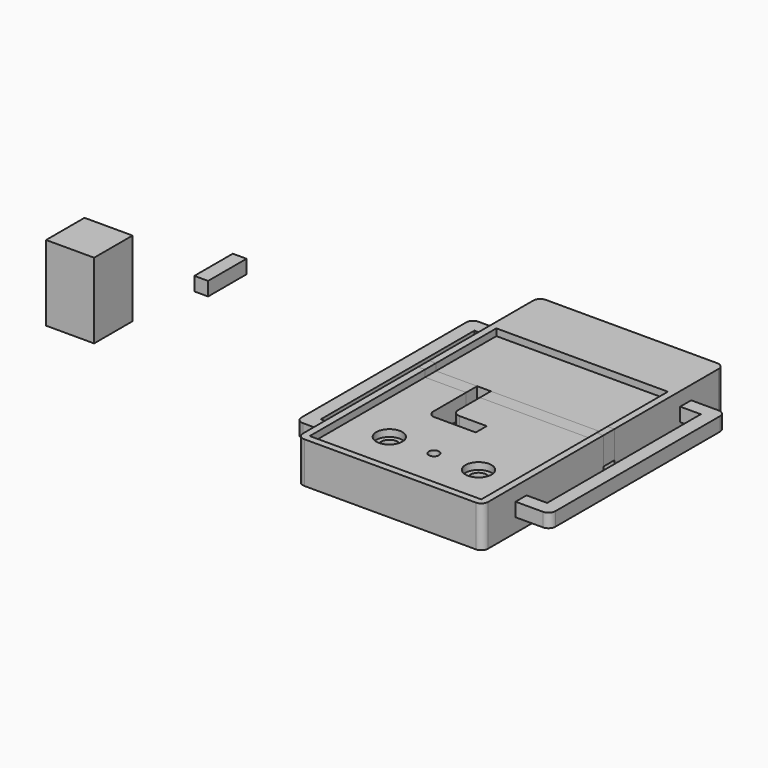
from build123d import *

# Parameters (mm, degrees)
F1_DEPTH  = 6
F0_R      = 1.9
F0_R_2    = 0.75
F2_DEPTH  = 5
F3_START  = 2
F3_DEPTH  = 2
F4_START  = 2
F0_W      = 1
F0_H      = 2
F4_DEPTH  = 4
F5_START  = 2.5
F0_W_2    = 6
F5_DEPTH  = 2.5
F0_W_3    = 17
F6_DEPTH  = 2
F0_R_3    = 1.2
F7_DEPTH  = 4
F8_W      = 2
F8_H      = 7
F9_DEPTH  = 2
F8_W_2    = 7
F10_DEPTH = 9


with BuildPart() as f1:
    # F0 (on Top) → F1 (new body)
    with BuildSketch(Plane.XY):
        with BuildLine():
            Line((12.5, 0), (0, 0))
            Line((0, 0), (-12.5, 0))
            Line((-12.5, 0), (-12.5, 21))
            Line((-12.5, 21), (-13.5, 21))
            Line((-13.5, 21), (-13.5, 7))
            Line((-13.5, 7), (-13.5, 5))
            Line((-13.5, 5), (-13.5, 0))
            ThreePointArc((-13.5, 0), (-13.2071067812, -0.7071067812), (-12.5, -1))
            Line((-12.5, -1), (0, -1))
            Line((0, -1), (12.5, -1))
            ThreePointArc((12.5, -1), (13.2071067812, -0.7071067812), (13.5, 0))
            Line((13.5, 0), (13.5, 5))
            Line((13.5, 5), (13.5, 7))
            Line((13.5, 7), (13.5, 21))
            Line((13.5, 21), (12.5, 21))
            Line((12.5, 21), (12.5, 0))
        make_face()
    extrude(amount=F1_DEPTH)


with BuildPart() as f1b:
    # F0 (on Top) → F1, piece 2 (new body)
    with BuildSketch(Plane.XY):
        with BuildLine():
            Line((-13.5, 23), (-12.5, 23))
            Line((-12.5, 23), (-12.5, 34))
            Line((-12.5, 34), (0, 34))
            Line((0, 34), (12.5, 34))
            Line((12.5, 34), (12.5, 23))
            Line((12.5, 23), (13.5, 23))
            Line((13.5, 23), (13.5, 35))
            Line((13.5, 35), (13.5, 37))
            Line((13.5, 37), (13.5, 42))
            ThreePointArc((13.5, 42), (13.2071067812, 42.7071067812), (12.5, 43))
            Line((12.5, 43), (0, 43))
            Line((0, 43), (-12.5, 43))
            ThreePointArc((-12.5, 43), (-13.2071067812, 42.7071067812), (-13.5, 42))
            Line((-13.5, 42), (-13.5, 37))
            Line((-13.5, 37), (-13.5, 35))
            Line((-13.5, 35), (-13.5, 23))
        make_face()
    extrude(amount=F1_DEPTH)

    # F0 (on Top) → F2, piece 2 (join)
    with BuildSketch(Plane.XY):
        Polygon((-12.5, 34), (-12.5, 23), (-6.5, 23), (-4.5, 23), (12.5, 23), (12.5, 34), (0, 34), align=None)
    extrude(amount=F2_DEPTH)


with BuildPart() as f2:
    # F0 (on Top) → F2 (new body)
    with BuildSketch(Plane.XY):
        with BuildLine():
            Line((-12.5, 0), (0, 0))
            Line((0, 0), (12.5, 0))
            Line((12.5, 0), (12.5, 21))
            Line((12.5, 21), (-4.5, 21))
            Line((-4.5, 21), (-4.5, 17))
            ThreePointArc((-4.5, 17), (-4.2071067812, 16.2928932188), (-3.5, 16))
            Line((-3.5, 16), (0.5, 16))
            Line((0.5, 16), (0.5, 14))
            Line((0.5, 14), (-2.5, 14))
            Line((-2.5, 14), (-5.5, 14))
            ThreePointArc((-5.5, 14), (-6.2071067812, 14.2928932188), (-6.5, 15))
            Line((-6.5, 15), (-6.5, 21))
            Line((-6.5, 21), (-12.5, 21))
            Line((-12.5, 21), (-12.5, 0))
        make_face()
        with Locations((-6.5, 7)):
            Circle(F0_R, mode=Mode.SUBTRACT)
        with Locations((0, 7)):
            Circle(F0_R_2, mode=Mode.SUBTRACT)
        with Locations((6.5, 7)):
            Circle(F0_R, mode=Mode.SUBTRACT)
    extrude(amount=F2_DEPTH)

    # F0 (on Top) → F7 (join)
    with BuildSketch(Plane.XY):
        with Locations((-6.5, 7)):
            Circle(F0_R)
        with Locations((-6.5, 7)):
            Circle(F0_R_3, mode=Mode.SUBTRACT)
        with Locations((6.5, 7)):
            Circle(F0_R)
        with Locations((6.5, 7)):
            Circle(F0_R_3, mode=Mode.SUBTRACT)
    extrude(amount=F7_DEPTH)


with BuildPart() as f3:
    # F0 (on Top) → F3 (new body)
    with BuildSketch(Plane.XY.offset(F3_START)):
        with BuildLine():
            Line((-13.5, 5), (-13.5, 7))
            Line((-13.5, 7), (-16.5, 7))
            Line((-16.5, 7), (-16.5, 35))
            Line((-16.5, 35), (-13.5, 35))
            Line((-13.5, 35), (-13.5, 37))
            Line((-13.5, 37), (-17.5, 37))
            ThreePointArc((-17.5, 37), (-18.2071067812, 36.7071067812), (-18.5, 36))
            Line((-18.5, 36), (-18.5, 6))
            ThreePointArc((-18.5, 6), (-18.2071067812, 5.2928932188), (-17.5, 5))
            Line((-17.5, 5), (-13.5, 5))
        make_face()
    extrude(amount=F3_DEPTH)


with BuildPart() as f3b:
    # F0 (on Top) → F3, piece 2 (new body)
    with BuildSketch(Plane.XY.offset(F3_START)):
        with BuildLine():
            Line((16.5, 7), (13.5, 7))
            Line((13.5, 7), (13.5, 5))
            Line((13.5, 5), (17.5, 5))
            ThreePointArc((17.5, 5), (18.2071067812, 5.2928932188), (18.5, 6))
            Line((18.5, 6), (18.5, 36))
            ThreePointArc((18.5, 36), (18.2071067812, 36.7071067812), (17.5, 37))
            Line((17.5, 37), (13.5, 37))
            Line((13.5, 37), (13.5, 35))
            Line((13.5, 35), (16.5, 35))
            Line((16.5, 35), (16.5, 7))
        make_face()
    extrude(amount=F3_DEPTH)


with BuildPart() as f4:
    # F0 (on Top) → F4 (new body)
    with BuildSketch(Plane.XY.offset(F4_START)):
        with Locations((-13, 22)):
            Rectangle(F0_W, F0_H)
    extrude(amount=F4_DEPTH)


with BuildPart() as f4b:
    # F0 (on Top) → F4, piece 2 (new body)
    with BuildSketch(Plane.XY.offset(F4_START)):
        with Locations((13, 22)):
            Rectangle(F0_W, F0_H)
    extrude(amount=F4_DEPTH)


with BuildPart() as f5:
    # F0 (on Top) → F5 (new body)
    with BuildSketch(Plane.XY.offset(F5_START)):
        with Locations((-9.5, 22)):
            Rectangle(F0_W_2, F0_H)
    extrude(amount=F5_DEPTH)


with BuildPart() as f5b:
    # F0 (on Top) → F5, piece 2 (new body)
    with BuildSketch(Plane.XY.offset(F5_START)):
        with Locations((4, 22)):
            Rectangle(F0_W_3, F0_H)
    extrude(amount=F5_DEPTH)


with BuildPart() as f6:
    # F0 (on Top) → F6 (new body)
    with BuildSketch(Plane.XY):
        with BuildLine():
            Line((-4.5, 21), (-6.5, 21))
            Line((-6.5, 21), (-6.5, 15))
            ThreePointArc((-6.5, 15), (-6.2071067812, 14.2928932188), (-5.5, 14))
            Line((-5.5, 14), (-2.5, 14))
            Line((-2.5, 14), (0.5, 14))
            Line((0.5, 14), (0.5, 16))
            Line((0.5, 16), (-3.5, 16))
            ThreePointArc((-3.5, 16), (-4.2071067812, 16.2928932188), (-4.5, 17))
            Line((-4.5, 17), (-4.5, 21))
        make_face()
    extrude(amount=F6_DEPTH)


with BuildPart() as f9:
    # F8 (on Top) → F9 (new body)
    with BuildSketch(Plane.XY):
        with Locations((-51.2206767944, 32.1291023865)):
            Rectangle(F8_W, F8_H)
    extrude(amount=F9_DEPTH)


with BuildPart() as f9b:
    # F8 (on Top) → F9, piece 2 (new body)
    with BuildSketch(Plane.XY):
        with Locations((-56.6243078709, 14.9900683984)):
            Rectangle(F8_W_2, F8_H)
    extrude(amount=F9_DEPTH)

    # F10 (add): a face of the model
    f10_faces = [f9b.faces().sort_by_distance(p)[0] for p in [
        (-56.6243078709, 14.9900683984, 2),
    ]]
    extrude(f10_faces, amount=F10_DEPTH)


solid = Compound([f1.part, f1b.part, f2.part, f3.part, f3b.part, f4.part, f4b.part, f5.part, f5b.part, f6.part, f9.part, f9b.part])
